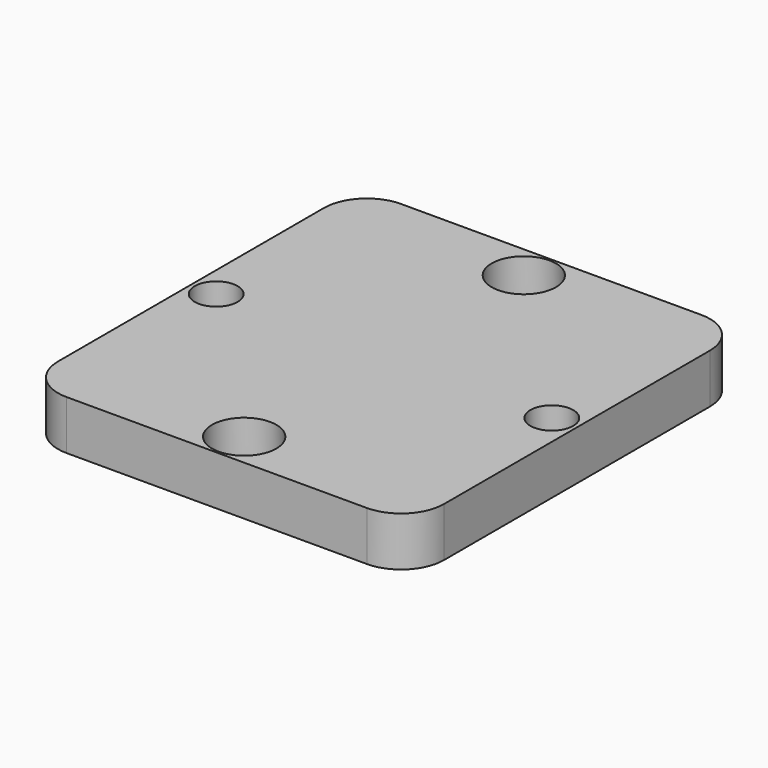
from build123d import *

# Parameters (mm, degrees)
F0_W     = 45.72
F0_H     = 49.53
F1_DEPTH = 5.842
F2_R     = 2.54
F3_DEPTH = 25.4
F4_R     = 3.81
F5_DEPTH = 4.064
F6_R     = 2.54
F7_DEPTH = 25.4
F8_R     = 5.08


# Not quite as in the source:
# - a feature names something its author has since deleted; it is built from what else it names


with BuildPart() as f1:
    # F0 (on Top) → F1 (new body)
    with BuildSketch(Plane.XY):
        Rectangle(F0_W, F0_H)
    extrude(amount=F1_DEPTH)

    # F2 (on face) → F3 (cut)
    with BuildSketch(Plane.XY.offset(5.842)):
        with Locations((-19.8755, 0)):
            Circle(F2_R)
        with Locations((19.8755, 0)):
            Circle(F2_R)
    extrude(amount=-F3_DEPTH, mode=Mode.SUBTRACT)

    # F4 (on face) → F5 (cut)
    with BuildSketch(Plane.XY.offset(5.842)):
        with Locations((0, 20.701)):
            Circle(F4_R)
        with Locations((0, -20.701)):
            Circle(F4_R)
    extrude(amount=-F5_DEPTH, mode=Mode.SUBTRACT)

    # F6 (on face) → F7 (cut)
    with BuildSketch(Plane.XY.offset(5.842)):
        with Locations((0, 20.701)):
            Circle(F6_R)
        with Locations((0, -20.701)):
            Circle(F6_R)
    extrude(amount=-F7_DEPTH, mode=Mode.SUBTRACT)

    # F8
    f8_edges = [f1.edges().sort_by_distance(p)[0] for p in [
        (-22.86, 24.765, 2.921),
        (-22.86, -24.765, 2.921),
        (22.86, -24.765, 2.921),
        (22.86, 24.765, 2.921),
    ]]
    fillet(f8_edges, radius=F8_R)


solid = f1.part
